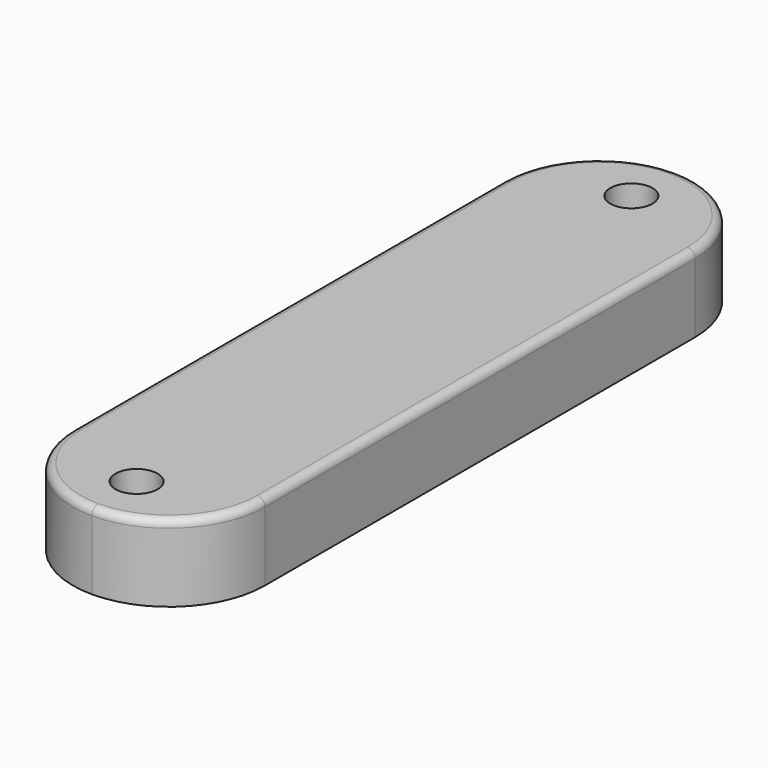
from build123d import *

# Parameters (mm, degrees)
F0_W     = 25
F0_H     = 95
F0_R     = 2.75
F1_DEPTH = 10
F2_R     = 12.49999
F3_R     = 1
F4_W     = 15
F4_H     = 70
F5_DEPTH = 6


# Not quite as in the source:
# - a fillet or chamfer is up to 0.001 mm smaller than in the source, because OpenCascade refuses the exact size


with BuildPart() as f1:
    # F0 (on Top) → F1 (new body)
    with BuildSketch(Plane.XY):
        with Locations((12.5, 47.5)):
            Rectangle(F0_W, F0_H)
        with Locations((12.5, 7.25)):
            Circle(F0_R, mode=Mode.SUBTRACT)
        with Locations((12.5, 87.75)):
            Circle(F0_R, mode=Mode.SUBTRACT)
    extrude(amount=F1_DEPTH)

    # F2 (radius 12.5 in the source; OpenCascade refuses exactly that, so slightly less here)
    f2_edges = [f1.edges().sort_by_distance(p)[0] for p in [
        (25, 95, 5),
        (0, 95, 5),
        (25, 0, 5),
        (0, 0, 5),
    ]]
    fillet(f2_edges, radius=F2_R)

    # F3
    f3_edges = [f1.edges().sort_by_distance(p)[0] for p in [
        (25, 47.5, 10),
        (0, 47.5, 10),
        (12.5, 95, 10),
        (21.338838, 91.338838, 10),
        (3.661162, 91.338838, 10),
        (21.338838, 3.661162, 10),
        (12.5, 0, 10),
        (3.661162, 3.661162, 10),
    ]]
    fillet(f3_edges, radius=F3_R)

    # F4 (on face) → F5 (cut)
    with BuildSketch(Plane(origin=(0, 0, 0), x_dir=(1, 0, 0), z_dir=(0, 0, -1))):
        with Locations((12.5, -47.5)):
            Rectangle(F4_W, F4_H)
    extrude(amount=-F5_DEPTH, mode=Mode.SUBTRACT)


solid = f1.part
